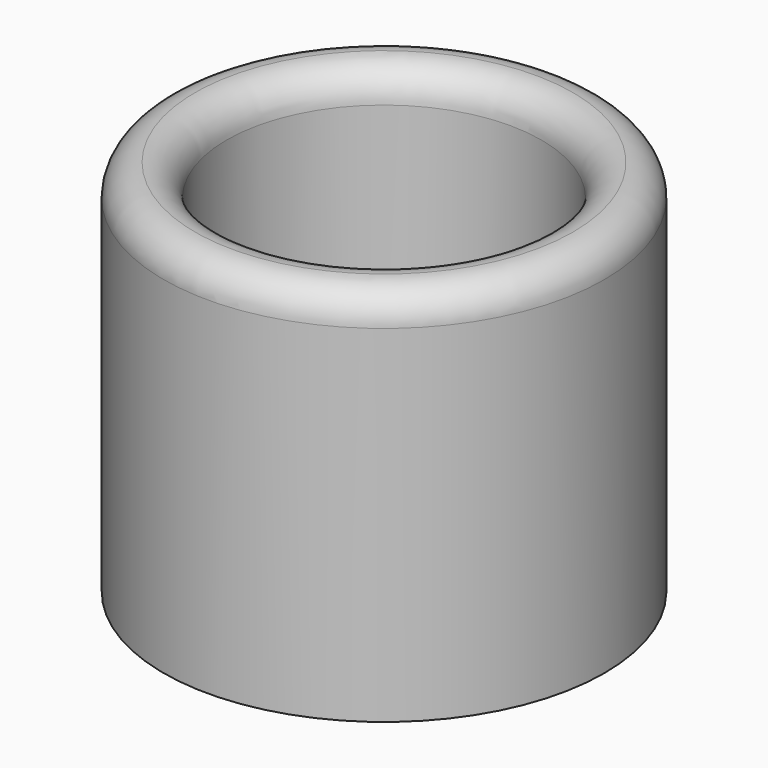
from build123d import *

# Parameters (mm, degrees)
F2_R     = 70
F3_DEPTH = 20
F4_R     = 70
F4_R_2   = 50
F5_DEPTH = 100
F6_R     = 9.99999


# Not quite as in the source:
# - a fillet or chamfer is up to 0.001 mm smaller than in the source, because OpenCascade refuses the exact size


with BuildPart() as f3:
    # F2 (on Top) → F3 (new body)
    with BuildSketch(Plane.XY):
        Circle(F2_R)
    extrude(amount=F3_DEPTH)

    # F4 (on face) → F5 (join)
    with BuildSketch(Plane.XY.offset(20)):
        Circle(F4_R)
        Circle(F4_R_2, mode=Mode.SUBTRACT)
    extrude(amount=F5_DEPTH)

    # F6 (radius 10 in the source; OpenCascade refuses exactly that, so slightly less here)
    f6_edges = [f3.edges().sort_by_distance(p)[0] for p in [
        (-50, 0, 120),
        (-70, 0, 120),
    ]]
    fillet(f6_edges, radius=F6_R)


solid = f3.part
